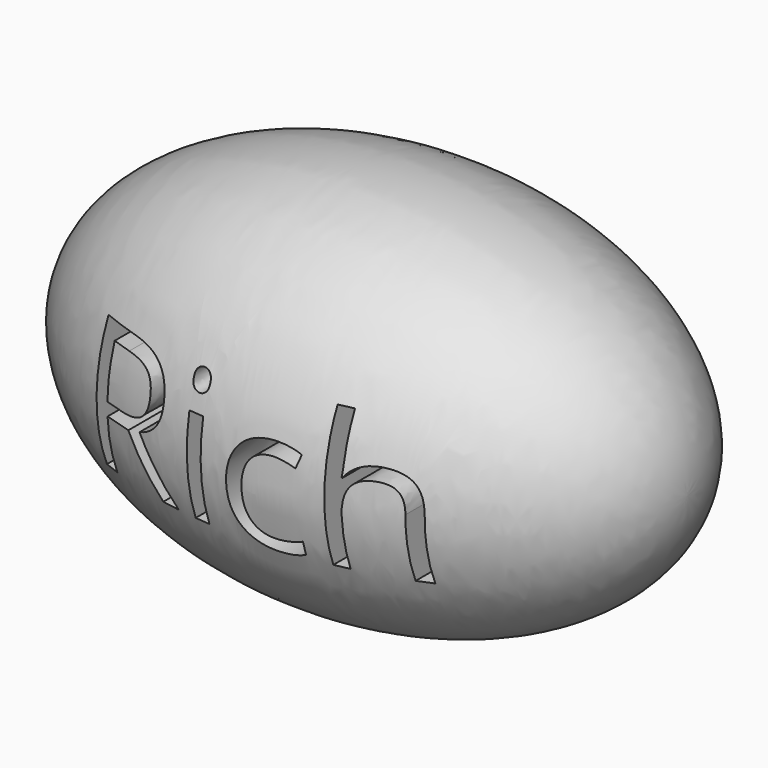
from build123d import *

# Parameters (mm, degrees)
F2_TEXT_SIZE = 78.0604709014
F3_DEPTH     = 226.9152998924


# Not quite as in the source:
# - a feature of the source that left no trace in its solid (it failed there, or was rolled back) is left out
# - Text() gives the source's letters only with a copy of the font that has no kerning and outlines rounded to 1/6400 em; it was checked with that copy


with BuildPart() as f1:
    # F0 (on Front) → F1 (revolve)
    with BuildSketch(Plane.XZ):
        with BuildLine():
            Line((-129.1410326958, 0), (129.1410326958, 0))
            add(Edge.make_bspline(
                [(129.1410326958, 0), (129.1410326958, 79.9738026991), (0, 79.9738026991), (-129.1410326958, 79.9738026991), (-129.1410326958, 0)],
                knots=[0, 0, 0, 1.5707963268, 1.5707963268, 3.1415926536, 3.1415926536, 3.1415926536], degree=2, weights=[1, 0.7071067812, 1, 0.7071067812, 1]))
        make_face()
    revolve(axis=Axis((0, 0, 0), (1, 0, 0)))


with BuildPart() as f3:
    # F2 (on Front) → F3 (new body)
    with BuildSketch(Plane.XZ):
        with Locations(Location((-75.9451526441, -26.9325445426), (0, 0, -0.0163849173))):
            Text('Rich', F2_TEXT_SIZE, font='Open Sans', text_align=(TextAlign.LEFT, TextAlign.BOTTOM))
    extrude(amount=F3_DEPTH)


with BuildPart() as f1_1:
    add(f1.part)

    # F4: cut F3
    add(f3.part, mode=Mode.SUBTRACT)


solid = f1_1.part
